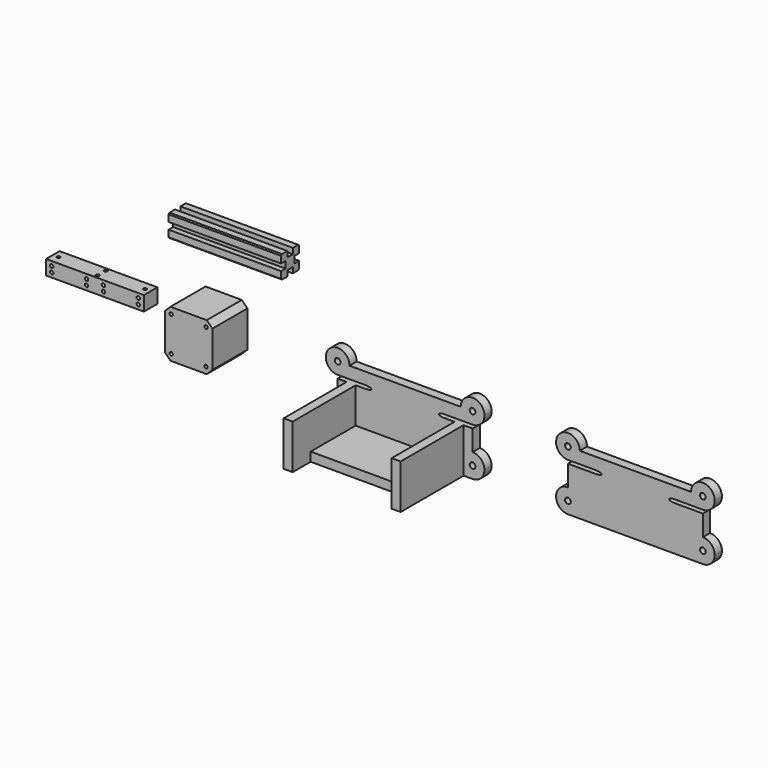
from build123d import *

# Parameters (mm, degrees)
F0_W      = 87
F0_H      = 13
F1_DEPTH  = 15
F3_DEPTH  = 25
F5_DEPTH  = 25
F7_DEPTH  = 39
F8_SIZE   = 5
F9_W      = 20
F9_H      = 20
F10_DEPTH = 100
F11_SIZE  = 1
F12_W     = 3
F12_H     = 5
F13_DEPTH = 148.2
F14_W     = 2.55
F14_H     = 15.5
F14_H_2   = 3
F15_DEPTH = 8
F18_DEPTH = 70
F19_W     = 88
F19_H     = 8
F20_DEPTH = 20


with BuildPart() as f1:
    # F0 (on Front) → F1 (new body)
    with BuildSketch(Plane.XZ):
        with Locations((-28.7405982092, 21.2712910548)):
            Rectangle(F0_W, F0_H)
    extrude(amount=F1_DEPTH)

    # F2 (on face) → F3 (cut)
    with BuildSketch(Plane.XZ.offset(15)):
        with BuildLine():
            ThreePointArc((-65.7405982092, 23.7712910548), (-66.1799380374, 24.8319512266), (-67.2405982092, 25.2712910548))
            Line((-67.2405982092, 25.2712910548), (-67.2405982092, 23.7712910548))
            Line((-67.2405982092, 23.7712910548), (-67.2405982092, 22.2712910548))
            ThreePointArc((-67.2405982092, 22.2712910548), (-66.1799380374, 22.710630883), (-65.7405982092, 23.7712910548))
        make_face()
        with BuildLine():
            Line((-67.2405982092, 23.7712910548), (-67.2405982092, 25.2712910548))
            ThreePointArc((-67.2405982092, 25.2712910548), (-68.7405982092, 23.7712910548), (-67.2405982092, 22.2712910548))
            Line((-67.2405982092, 22.2712910548), (-67.2405982092, 23.7712910548))
        make_face()
        with BuildLine():
            ThreePointArc((-67.2405982092, 20.2712910548), (-68.7405982092, 18.7712910548), (-67.2405982092, 17.2712910548))
            Line((-67.2405982092, 17.2712910548), (-67.2405982092, 18.7712910548))
            Line((-67.2405982092, 18.7712910548), (-67.2405982092, 20.2712910548))
        make_face()
        with BuildLine():
            Line((-67.2405982092, 18.7712910548), (-67.2405982092, 17.2712910548))
            ThreePointArc((-67.2405982092, 17.2712910548), (-66.1799380374, 17.710630883), (-65.7405982092, 18.7712910548))
            ThreePointArc((-65.7405982092, 18.7712910548), (-66.1799380374, 19.8319512266), (-67.2405982092, 20.2712910548))
            Line((-67.2405982092, 20.2712910548), (-67.2405982092, 18.7712910548))
        make_face()
        with BuildLine():
            Line((-34.7405982092, 23.7712910548), (-36.2405982092, 23.7712910548))
            Line((-36.2405982092, 23.7712910548), (-36.2405982092, 22.2712910548))
            ThreePointArc((-36.2405982092, 22.2712910548), (-35.1799380374, 22.710630883), (-34.7405982092, 23.7712910548))
        make_face()
        with BuildLine():
            Line((-36.2405982092, 23.7712910548), (-36.2405982092, 25.2712910548))
            ThreePointArc((-36.2405982092, 25.2712910548), (-37.7405982092, 23.7712910548), (-36.2405982092, 22.2712910548))
            Line((-36.2405982092, 22.2712910548), (-36.2405982092, 23.7712910548))
        make_face()
        with BuildLine():
            ThreePointArc((-34.7405982092, 23.7712910548), (-35.1799380374, 24.8319512266), (-36.2405982092, 25.2712910548))
            Line((-36.2405982092, 25.2712910548), (-36.2405982092, 23.7712910548))
            Line((-36.2405982092, 23.7712910548), (-34.7405982092, 23.7712910548))
        make_face()
        with BuildLine():
            ThreePointArc((-34.7405982092, 18.7712910548), (-35.1799380374, 19.8319512266), (-36.2405982092, 20.2712910548))
            ThreePointArc((-36.2405982092, 20.2712910548), (-37.301258381, 17.710630883), (-34.7405982092, 18.7712910548))
        make_face()
        with BuildLine():
            ThreePointArc((-19.7405982092, 23.7712910548), (-21.2405982092, 25.2712910548), (-22.7405982092, 23.7712910548))
            Line((-22.7405982092, 23.7712910548), (-21.2405982092, 23.7712910548))
            Line((-21.2405982092, 23.7712910548), (-21.2405982092, 22.2712910548))
            ThreePointArc((-21.2405982092, 22.2712910548), (-20.1799380374, 22.710630883), (-19.7405982092, 23.7712910548))
        make_face()
        with BuildLine():
            Line((-21.2405982092, 23.7712910548), (-22.7405982092, 23.7712910548))
            ThreePointArc((-22.7405982092, 23.7712910548), (-22.301258381, 22.710630883), (-21.2405982092, 22.2712910548))
            Line((-21.2405982092, 22.2712910548), (-21.2405982092, 23.7712910548))
        make_face()
        with BuildLine():
            Line((-21.2405982092, 18.7712910548), (-21.2405982092, 20.2712910548))
            ThreePointArc((-21.2405982092, 20.2712910548), (-22.301258381, 17.710630883), (-19.7405982092, 18.7712910548))
            Line((-19.7405982092, 18.7712910548), (-21.2405982092, 18.7712910548))
        make_face()
        with BuildLine():
            ThreePointArc((-19.7405982092, 18.7712910548), (-20.1799380374, 19.8319512266), (-21.2405982092, 20.2712910548))
            Line((-21.2405982092, 20.2712910548), (-21.2405982092, 18.7712910548))
            Line((-21.2405982092, 18.7712910548), (-19.7405982092, 18.7712910548))
        make_face()
        with BuildLine():
            Line((9.7594017908, 18.7712910548), (8.2594017908, 18.7712910548))
            ThreePointArc((8.2594017908, 18.7712910548), (9.7594017908, 17.2712910548), (11.2594017908, 18.7712910548))
            ThreePointArc((11.2594017908, 18.7712910548), (10.8200619626, 19.8319512266), (9.7594017908, 20.2712910548))
            Line((9.7594017908, 20.2712910548), (9.7594017908, 18.7712910548))
        make_face()
        with BuildLine():
            ThreePointArc((9.7594017908, 20.2712910548), (8.698741619, 19.8319512266), (8.2594017908, 18.7712910548))
            Line((8.2594017908, 18.7712910548), (9.7594017908, 18.7712910548))
            Line((9.7594017908, 18.7712910548), (9.7594017908, 20.2712910548))
        make_face()
        with BuildLine():
            ThreePointArc((11.2594017908, 23.7712910548), (8.698741619, 24.8319512266), (9.7594017908, 22.2712910548))
            ThreePointArc((9.7594017908, 22.2712910548), (10.8200619626, 22.710630883), (11.2594017908, 23.7712910548))
        make_face()
    extrude(amount=-F3_DEPTH, mode=Mode.SUBTRACT)

    # F4 (on face) → F5 (cut)
    with BuildSketch(Plane.XY.offset(27.7712910548)):
        with BuildLine():
            Line((-68.7405982092, -7.5), (-67.2405982092, -7.5))
            Line((-67.2405982092, -7.5), (-65.7405982092, -7.5))
            ThreePointArc((-65.7405982092, -7.5), (-67.2405982092, -6), (-68.7405982092, -7.5))
        make_face()
        with BuildLine():
            Line((-65.7405982092, -7.5), (-67.2405982092, -7.5))
            Line((-67.2405982092, -7.5), (-68.7405982092, -7.5))
            ThreePointArc((-68.7405982092, -7.5), (-67.2405982092, -9), (-65.7405982092, -7.5))
        make_face()
        with BuildLine():
            ThreePointArc((-28.7405982092, -1.5), (-30.2405982092, -3), (-28.7405982092, -4.5))
            Line((-28.7405982092, -4.5), (-28.7405982092, -3))
            Line((-28.7405982092, -3), (-28.7405982092, -1.5))
        make_face()
        with BuildLine():
            Line((-28.7405982092, -3), (-28.7405982092, -4.5))
            ThreePointArc((-28.7405982092, -4.5), (-27.6799380374, -4.0606601718), (-27.2405982092, -3))
            ThreePointArc((-27.2405982092, -3), (-27.6799380374, -1.9393398282), (-28.7405982092, -1.5))
            Line((-28.7405982092, -1.5), (-28.7405982092, -3))
        make_face()
        with BuildLine():
            ThreePointArc((11.2594017908, -7.5), (9.7594017908, -6), (8.2594017908, -7.5))
            Line((8.2594017908, -7.5), (9.7594017908, -7.5))
            Line((9.7594017908, -7.5), (11.2594017908, -7.5))
        make_face()
        with BuildLine():
            Line((9.7594017908, -7.5), (8.2594017908, -7.5))
            ThreePointArc((8.2594017908, -7.5), (9.7594017908, -9), (11.2594017908, -7.5))
            Line((11.2594017908, -7.5), (9.7594017908, -7.5))
        make_face()
        with BuildLine():
            ThreePointArc((-27.2405982092, -12), (-27.6799380374, -10.9393398282), (-28.7405982092, -10.5))
            Line((-28.7405982092, -10.5), (-28.7405982092, -12))
            Line((-28.7405982092, -12), (-28.7405982092, -13.5))
            ThreePointArc((-28.7405982092, -13.5), (-27.6799380374, -13.0606601718), (-27.2405982092, -12))
        make_face()
        with BuildLine():
            Line((-28.7405982092, -12), (-28.7405982092, -10.5))
            ThreePointArc((-28.7405982092, -10.5), (-30.2405982092, -12), (-28.7405982092, -13.5))
            Line((-28.7405982092, -13.5), (-28.7405982092, -12))
        make_face()
    extrude(amount=-F5_DEPTH, mode=Mode.SUBTRACT)


with BuildPart() as f7:
    # F6 (on Front) → F7 (new body)
    with BuildSketch(Plane.XZ):
        with BuildLine():
            Line((58.2019463181, 42.3), (52.5519463181, 42.3))
            Line((52.5519463181, 42.3), (52.5519463181, 36.65))
            Line((52.5519463181, 36.65), (56.7019463181, 36.65))
            ThreePointArc((56.7019463181, 36.65), (57.1412861464, 37.7106601718), (58.2019463181, 38.15))
            Line((58.2019463181, 38.15), (58.2019463181, 42.3))
        make_face()
        with BuildLine():
            Line((94.8519463181, 42.3), (58.2019463181, 42.3))
            Line((58.2019463181, 42.3), (58.2019463181, 38.15))
            ThreePointArc((58.2019463181, 38.15), (59.2626064899, 37.7106601718), (59.7019463181, 36.65))
            Line((59.7019463181, 36.65), (87.7019463181, 36.65))
            ThreePointArc((87.7019463181, 36.65), (89.2019463181, 38.15), (90.7019463181, 36.65))
            Line((90.7019463181, 36.65), (94.8519463181, 36.65))
            Line((94.8519463181, 36.65), (94.8519463181, 42.3))
        make_face()
        with BuildLine():
            Line((56.7019463181, 36.65), (52.5519463181, 36.65))
            Line((52.5519463181, 36.65), (52.5519463181, 0))
            Line((52.5519463181, 0), (94.8519463181, 0))
            Line((94.8519463181, 0), (94.8519463181, 36.65))
            Line((94.8519463181, 36.65), (90.7019463181, 36.65))
            ThreePointArc((90.7019463181, 36.65), (90.2626064899, 35.5893398282), (89.2019463181, 35.15))
            Line((89.2019463181, 35.15), (89.2019463181, 7.15))
            ThreePointArc((89.2019463181, 7.15), (90.2626064899, 6.7106601718), (90.7019463181, 5.65))
            ThreePointArc((90.7019463181, 5.65), (89.2019463181, 4.15), (87.7019463181, 5.65))
            Line((87.7019463181, 5.65), (59.7019463181, 5.65))
            ThreePointArc((59.7019463181, 5.65), (57.1412861464, 4.5893398282), (58.2019463181, 7.15))
            Line((58.2019463181, 7.15), (58.2019463181, 35.15))
            ThreePointArc((58.2019463181, 35.15), (57.1412861464, 35.5893398282), (56.7019463181, 36.65))
        make_face()
        with BuildLine():
            Line((87.7019463181, 36.65), (59.7019463181, 36.65))
            ThreePointArc((59.7019463181, 36.65), (59.2626064899, 35.5893398282), (58.2019463181, 35.15))
            Line((58.2019463181, 35.15), (58.2019463181, 7.15))
            ThreePointArc((58.2019463181, 7.15), (59.2626064899, 6.7106601718), (59.7019463181, 5.65))
            Line((59.7019463181, 5.65), (87.7019463181, 5.65))
            ThreePointArc((87.7019463181, 5.65), (88.1412861464, 6.7106601718), (89.2019463181, 7.15))
            Line((89.2019463181, 7.15), (89.2019463181, 35.15))
            ThreePointArc((89.2019463181, 35.15), (88.1412861464, 35.5893398282), (87.7019463181, 36.65))
        make_face()
    extrude(amount=F7_DEPTH)

    # F8
    f8_edges = [f7.edges().sort_by_distance(p)[0] for p in [
        (52.551946, -19.5, 42.3),
        (94.851946, -19.5, 42.3),
        (52.551946, -19.5, 0),
        (94.851946, -19.5, 0),
    ]]
    chamfer(f8_edges, length=F8_SIZE)


with BuildPart() as f10:
    # F9 (on Right) → F10 (new body)
    with BuildSketch(Plane.YZ):
        with Locations((41.0009028763, 58.4589114785)):
            Rectangle(F9_W, F9_H)
    extrude(amount=F10_DEPTH)

    # F11
    f11_edges = [f10.edges().sort_by_distance(p)[0] for p in [
        (50, 31.000903, 68.458911),
        (50, 51.000903, 68.458911),
        (50, 31.000903, 48.458911),
        (50, 51.000903, 48.458911),
    ]]
    chamfer(f11_edges, length=F11_SIZE)

    # F12 (on face) → F13 (cut)
    with BuildSketch(Plane(origin=(0, 0, 0), x_dir=(0, -1, 0), z_dir=(-1, 0, 0))):
        with Locations((-42.5009028763, 50.9589114785)):
            Rectangle(F12_W, F12_H)
        with Locations((-39.5009028763, 50.9589114785)):
            Rectangle(F12_W, F12_H)
        with Locations((-42.5009028763, 65.9589114785)):
            Rectangle(F12_W, F12_H)
        with Locations((-39.5009028763, 65.9589114785)):
            Rectangle(F12_W, F12_H)
        Polygon((-46.0009028763, 61.4589114785), (-51.0009028763, 61.4589114785), (-51.0009028763, 58.4589114785), (-51.0009028763, 55.4589114785), (-46.0009028763, 55.4589114785), align=None)
        Polygon((-31.0009028763, 61.4589114785), (-36.0009028763, 61.4589114785), (-36.0009028763, 58.4589114785), (-36.0009028763, 55.4589114785), (-31.0009028763, 55.4589114785), align=None)
    extrude(amount=-F13_DEPTH, mode=Mode.SUBTRACT)


with BuildPart() as f15:
    # F14 (on Front) → F15 (new body)
    with BuildSketch(Plane.XZ):
        with BuildLine():
            ThreePointArc((178.9015343745, 27.2655571997), (181.4515343745, 29.8155571997), (184.0015343745, 27.2655571997))
            Line((184.0015343745, 27.2655571997), (192.0015343745, 27.2655571997))
            ThreePointArc((192.0015343745, 27.2655571997), (181.4515343745, 37.8155571997), (170.9015343745, 27.2655571997))
            Line((170.9015343745, 27.2655571997), (178.9015343745, 27.2655571997))
        make_face()
        with BuildLine():
            Line((192.0015343745, 27.2655571997), (184.0015343745, 27.2655571997))
            ThreePointArc((184.0015343745, 27.2655571997), (183.2546566665, 25.4624349077), (181.4515343745, 24.7155571997))
            Line((181.4515343745, 24.7155571997), (181.4515343745, 16.7155571997))
            ThreePointArc((181.4515343745, 16.7155571997), (188.911510916, 19.8055806582), (192.0015343745, 27.2655571997))
        make_face()
        with BuildLine():
            Line((181.4515343745, 16.7155571997), (181.4515343745, 24.7155571997))
            ThreePointArc((181.4515343745, 24.7155571997), (179.6484120825, 25.4624349077), (178.9015343745, 27.2655571997))
            Line((178.9015343745, 27.2655571997), (170.9015343745, 27.2655571997))
            ThreePointArc((170.9015343745, 27.2655571997), (173.991557833, 19.8055806582), (181.4515343745, 16.7155571997))
        make_face()
        with BuildLine():
            Line((241.4515343745, 27.2655571997), (192.0015343745, 27.2655571997))
            ThreePointArc((192.0015343745, 27.2655571997), (188.911510916, 19.8055806582), (181.4515343745, 16.7155571997))
            Line((181.4515343745, 16.7155571997), (206.4515343745, 16.7155571997))
            Line((206.4515343745, 16.7155571997), (211.4515343745, 16.7155571997))
            Line((211.4515343745, 16.7155571997), (241.4515343745, 16.7155571997))
            Line((241.4515343745, 16.7155571997), (241.4515343745, 27.2655571997))
        make_face()
        with BuildLine():
            Line((282.7265343745, 27.2655571997), (241.4515343745, 27.2655571997))
            Line((241.4515343745, 27.2655571997), (241.4515343745, 16.7155571997))
            Line((241.4515343745, 16.7155571997), (276.4515343745, 16.7155571997))
            Line((276.4515343745, 16.7155571997), (290.9015343745, 16.7155571997))
            Line((290.9015343745, 16.7155571997), (301.4515343745, 16.7155571997))
            ThreePointArc((301.4515343745, 16.7155571997), (293.991557833, 19.8055806582), (290.9015343745, 27.2655571997))
            Line((290.9015343745, 27.2655571997), (282.7265343745, 27.2655571997))
        make_face()
        Polygon((184.0015343745, 13.7155571997), (181.4515343745, 13.7155571997), (181.4515343745, -1.7844428003), (206.4515343745, -1.7844428003), (211.4515343745, -1.7844428003), (211.4515343745, 13.7155571997), (206.4515343745, 13.7155571997), (192.0015343745, 13.7155571997), align=None)
        with BuildLine():
            Line((211.4515343745, 16.7155571997), (206.4515343745, 16.7155571997))
            add(Edge.make_bspline(
                [(211.4515343745, 15.2155571997), (211.4515343745, 16.7155571997), (206.4515343745, 16.7155571997)],
                knots=[0, 0, 0, 1.5707963268, 1.5707963268, 1.5707963268], degree=2, weights=[1, 0.7071067812, 1]))
            Line((211.4515343745, 15.2155571997), (211.4515343745, 16.7155571997))
        make_face()
        Polygon((241.4515343745, 13.7155571997), (241.4515343745, 16.7155571997), (211.4515343745, 16.7155571997), (211.4515343745, 15.2155571997), (211.4515343745, 13.7155571997), align=None)
        with BuildLine():
            Line((276.4515343745, 16.7155571997), (241.4515343745, 16.7155571997))
            Line((241.4515343745, 16.7155571997), (241.4515343745, 13.7155571997))
            Line((241.4515343745, 13.7155571997), (276.4515343664, 13.7155571997))
            add(Edge.make_bspline(
                [(271.4515343745, 15.2155571997), (271.4515343745, 13.7155572022), (276.4515343664, 13.7155571997)],
                knots=[0, 0, 0, 1.5707963252, 1.5707963252, 1.5707963252], degree=2, weights=[1, 0.7071067818, 1]))
            add(Edge.make_bspline(
                [(276.4515343745, 16.7155571997), (271.4515343745, 16.7155571997), (271.4515343745, 15.2155571997)],
                knots=[4.7123889804, 4.7123889804, 4.7123889804, 6.2831853072, 6.2831853072, 6.2831853072], degree=2, weights=[1, 0.7071067812, 1]))
        make_face()
        with BuildLine():
            Line((206.4515343745, -1.7844428003), (181.4515343745, -1.7844428003))
            Line((181.4515343745, -1.7844428003), (181.4515343745, -4.7844428003))
            Line((181.4515343745, -4.7844428003), (206.4515343745, -4.7844428003))
            add(Edge.make_bspline(
                [(206.4515343745, -1.7844428003), (201.4515343745, -1.7844428003), (201.4515343745, -3.2844428003), (201.4515343745, -4.7844428003), (206.4515343745, -4.7844428003)],
                knots=[1.5707963268, 1.5707963268, 1.5707963268, 3.1415926536, 3.1415926536, 4.7123889804, 4.7123889804, 4.7123889804], degree=2, weights=[1, 0.7071067812, 1, 0.7071067812, 1]))
        make_face()
        with BuildLine():
            Line((211.4515343745, 13.7155571997), (211.4515343745, 15.2155571997))
            add(Edge.make_bspline(
                [(206.4515343745, 13.7155571997), (211.4515343745, 13.7155571997), (211.4515343745, 15.2155571997)],
                knots=[4.7123889804, 4.7123889804, 4.7123889804, 6.2831853072, 6.2831853072, 6.2831853072], degree=2, weights=[1, 0.7071067812, 1]))
            Line((206.4515343745, 13.7155571997), (211.4515343745, 13.7155571997))
        make_face()
        with BuildLine():
            ThreePointArc((312.0015343745, 27.2655571997), (301.4515343745, 37.8155571997), (290.9015343745, 27.2655571997))
            ThreePointArc((290.9015343745, 27.2655571997), (293.991557833, 19.8055806582), (301.4515343745, 16.7155571997))
            ThreePointArc((301.4515343745, 16.7155571997), (308.911510916, 19.8055806582), (312.0015343745, 27.2655571997))
        make_face()
        with BuildLine():
            ThreePointArc((304.0015343745, 27.2655571997), (303.2546566665, 25.4624349077), (301.4515343745, 24.7155571997))
            ThreePointArc((301.4515343745, 24.7155571997), (299.6484120825, 29.0686794917), (304.0015343745, 27.2655571997))
        make_face(mode=Mode.SUBTRACT)
        Polygon((241.4515343745, 5.9655571997), (241.4515343745, 13.7155571997), (211.4515343745, 13.7155571997), (211.4515343745, -1.7844428003), (241.4515343745, -1.7844428003), align=None)
        Polygon((276.4515343664, 13.7155571997), (241.4515343745, 13.7155571997), (241.4515343745, 5.9655571997), (241.4515343745, -1.7844428003), (276.4515343745, -1.7844428003), (290.9015343745, -1.7844428003), (298.9015343745, -1.7844428003), (298.9015343745, 13.7155571997), (290.9015343745, 13.7155571997), align=None)
        with BuildLine():
            ThreePointArc((192.0015343745, -15.3344428003), (188.911510916, -7.8744662588), (181.4515343745, -4.7844428003))
            Line((181.4515343745, -4.7844428003), (181.4515343745, -12.7844428003))
            ThreePointArc((181.4515343745, -12.7844428003), (183.2546566665, -13.5313205083), (184.0015343745, -15.3344428003))
            Line((184.0015343745, -15.3344428003), (192.0015343745, -15.3344428003))
        make_face()
        with BuildLine():
            Line((206.4515343745, -4.7844428003), (181.4515343745, -4.7844428003))
            ThreePointArc((181.4515343745, -4.7844428003), (188.911510916, -7.8744662588), (192.0015343745, -15.3344428003))
            Line((192.0015343745, -15.3344428003), (241.4515343745, -15.3344428003))
            Line((241.4515343745, -15.3344428003), (241.4515343745, -4.7844428003))
            Line((241.4515343745, -4.7844428003), (211.4515343745, -4.7844428003))
            Line((211.4515343745, -4.7844428003), (206.4515343745, -4.7844428003))
        make_face()
        with BuildLine():
            Line((181.4515343745, -12.7844428003), (181.4515343745, -4.7844428003))
            ThreePointArc((181.4515343745, -4.7844428003), (173.991557833, -7.8744662588), (170.9015343745, -15.3344428003))
            Line((170.9015343745, -15.3344428003), (178.9015343745, -15.3344428003))
            ThreePointArc((178.9015343745, -15.3344428003), (179.6484120825, -13.5313205083), (181.4515343745, -12.7844428003))
        make_face()
        with BuildLine():
            Line((211.4515343745, -1.7844428003), (206.4515343745, -1.7844428003))
            add(Edge.make_bspline(
                [(211.4515343745, -3.2844428003), (211.4515343745, -1.7844428003), (206.4515343745, -1.7844428003)],
                knots=[0, 0, 0, 1.5707963268, 1.5707963268, 1.5707963268], degree=2, weights=[1, 0.7071067812, 1]))
            Line((211.4515343745, -3.2844428003), (211.4515343745, -1.7844428003))
        make_face()
        with BuildLine():
            add(Edge.make_bspline(
                [(211.4515343745, -3.2844428003), (211.4515343745, -1.7844428003), (206.4515343745, -1.7844428003)],
                knots=[0, 0, 0, 1.5707963268, 1.5707963268, 1.5707963268], degree=2, weights=[1, 0.7071067812, 1]))
            add(Edge.make_bspline(
                [(206.4515343745, -1.7844428003), (201.4515343745, -1.7844428003), (201.4515343745, -3.2844428003), (201.4515343745, -4.7844428003), (206.4515343745, -4.7844428003)],
                knots=[1.5707963268, 1.5707963268, 1.5707963268, 3.1415926536, 3.1415926536, 4.7123889804, 4.7123889804, 4.7123889804], degree=2, weights=[1, 0.7071067812, 1, 0.7071067812, 1]))
            add(Edge.make_bspline(
                [(206.4515343745, -4.7844428003), (211.4515343745, -4.7844428003), (211.4515343745, -3.2844428003)],
                knots=[4.7123889804, 4.7123889804, 4.7123889804, 6.2831853072, 6.2831853072, 6.2831853072], degree=2, weights=[1, 0.7071067812, 1]))
        make_face()
        with BuildLine():
            ThreePointArc((181.4515343745, -25.8844428003), (188.911510916, -22.7944193418), (192.0015343745, -15.3344428003))
            Line((192.0015343745, -15.3344428003), (184.0015343745, -15.3344428003))
            ThreePointArc((184.0015343745, -15.3344428003), (183.2546566665, -17.1375650923), (181.4515343745, -17.8844428003))
            Line((181.4515343745, -17.8844428003), (181.4515343745, -25.8844428003))
        make_face()
        with BuildLine():
            Line((241.4515343745, -15.3344428003), (192.0015343745, -15.3344428003))
            ThreePointArc((192.0015343745, -15.3344428003), (188.911510916, -22.7944193418), (181.4515343745, -25.8844428003))
            Line((181.4515343745, -25.8844428003), (192.0015343745, -25.8844428003))
            Line((192.0015343745, -25.8844428003), (241.4515343745, -25.8844428003))
            Line((241.4515343745, -25.8844428003), (241.4515343745, -15.3344428003))
        make_face()
        with BuildLine():
            Line((178.9015343745, -15.3344428003), (170.9015343745, -15.3344428003))
            ThreePointArc((170.9015343745, -15.3344428003), (173.991557833, -22.7944193418), (181.4515343745, -25.8844428003))
            Line((181.4515343745, -25.8844428003), (181.4515343745, -17.8844428003))
            ThreePointArc((181.4515343745, -17.8844428003), (179.6484120825, -17.1375650923), (178.9015343745, -15.3344428003))
        make_face()
        with BuildLine():
            add(Edge.make_bspline(
                [(206.4515343745, -4.7844428003), (211.4515343745, -4.7844428003), (211.4515343745, -3.2844428003)],
                knots=[4.7123889804, 4.7123889804, 4.7123889804, 6.2831853072, 6.2831853072, 6.2831853072], degree=2, weights=[1, 0.7071067812, 1]))
            Line((206.4515343745, -4.7844428003), (211.4515343745, -4.7844428003))
            Line((211.4515343745, -4.7844428003), (211.4515343745, -3.2844428003))
        make_face()
        Polygon((241.4515343745, -1.7844428003), (211.4515343745, -1.7844428003), (211.4515343745, -3.2844428003), (211.4515343745, -4.7844428003), (241.4515343745, -4.7844428003), align=None)
        with Locations((300.1765343745, 5.9655571997)):
            Rectangle(F14_W, F14_H)
        with BuildLine():
            Line((276.4515343745, -1.7844428003), (241.4515343745, -1.7844428003))
            Line((241.4515343745, -1.7844428003), (241.4515343745, -4.7844428003))
            Line((241.4515343745, -4.7844428003), (262.8303221703, -4.7844428003))
            Line((262.8303221703, -4.7844428003), (276.4515343745, -4.7844428003))
            add(Edge.make_bspline(
                [(271.4515343745, -3.2844428003), (271.4515343745, -4.7844428003), (276.4515343745, -4.7844428003)],
                knots=[0, 0, 0, 1.5707963268, 1.5707963268, 1.5707963268], degree=2, weights=[1, 0.7071067812, 1]))
            add(Edge.make_bspline(
                [(276.4515343745, -1.7844428003), (271.4515343745, -1.7844428003), (271.4515343745, -3.2844428003)],
                knots=[4.7123889804, 4.7123889804, 4.7123889804, 6.2831853072, 6.2831853072, 6.2831853072], degree=2, weights=[1, 0.7071067812, 1]))
        make_face()
        with BuildLine():
            Line((241.4515343745, -4.7844428003), (241.4515343745, -15.3344428003))
            Line((241.4515343745, -15.3344428003), (282.7265343745, -15.3344428003))
            Line((282.7265343745, -15.3344428003), (290.7265343745, -15.3344428003))
            Line((290.7265343745, -15.3344428003), (290.9015343745, -15.3344428003))
            ThreePointArc((290.9015343745, -15.3344428003), (293.1387430262, -8.8382900927), (298.9015343745, -5.0972556866))
            Line((298.9015343745, -5.0972556866), (298.9015343745, -4.7844428003))
            Line((298.9015343745, -4.7844428003), (276.4515343745, -4.7844428003))
            Line((276.4515343745, -4.7844428003), (262.8303221703, -4.7844428003))
            Line((262.8303221703, -4.7844428003), (241.4515343745, -4.7844428003))
        make_face()
        with BuildLine():
            Line((282.7265343745, -15.3344428003), (241.4515343745, -15.3344428003))
            Line((241.4515343745, -15.3344428003), (241.4515343745, -25.8844428003))
            Line((241.4515343745, -25.8844428003), (285.4515343745, -25.8844428003))
            Line((285.4515343745, -25.8844428003), (290.9015343745, -25.8844428003))
            Line((290.9015343745, -25.8844428003), (301.4515343745, -25.8844428003))
            ThreePointArc((301.4515343745, -25.8844428003), (300.1669768727, -25.8059475644), (298.9015343745, -25.5716299139))
            ThreePointArc((298.9015343745, -25.5716299139), (293.1387430262, -21.8305955078), (290.9015343745, -15.3344428003))
            Line((290.9015343745, -15.3344428003), (290.7265343745, -15.3344428003))
            Line((290.7265343745, -15.3344428003), (282.7265343745, -15.3344428003))
        make_face()
        with Locations((300.1765343745, -3.2844428003)):
            Rectangle(F14_W, F14_H_2)
        with BuildLine():
            Line((290.9015343745, -1.7844428003), (276.4515343745, -1.7844428003))
            add(Edge.make_bspline(
                [(276.4515343745, -4.7844428003), (281.4515343745, -4.7844428003), (281.4515343745, -3.2844428003), (281.4515343745, -1.7844428003), (276.4515343745, -1.7844428003)],
                knots=[1.5707963268, 1.5707963268, 1.5707963268, 3.1415926536, 3.1415926536, 4.7123889804, 4.7123889804, 4.7123889804], degree=2, weights=[1, 0.7071067812, 1, 0.7071067812, 1]))
            Line((276.4515343745, -4.7844428003), (298.9015343745, -4.7844428003))
            Line((298.9015343745, -4.7844428003), (298.9015343745, -1.7844428003))
            Line((298.9015343745, -1.7844428003), (290.9015343745, -1.7844428003))
        make_face()
        with BuildLine():
            add(Edge.make_bspline(
                [(276.4515343745, -4.7844428003), (281.4515343745, -4.7844428003), (281.4515343745, -3.2844428003), (281.4515343745, -1.7844428003), (276.4515343745, -1.7844428003)],
                knots=[1.5707963268, 1.5707963268, 1.5707963268, 3.1415926536, 3.1415926536, 4.7123889804, 4.7123889804, 4.7123889804], degree=2, weights=[1, 0.7071067812, 1, 0.7071067812, 1]))
            add(Edge.make_bspline(
                [(276.4515343745, -1.7844428003), (271.4515343745, -1.7844428003), (271.4515343745, -3.2844428003)],
                knots=[4.7123889804, 4.7123889804, 4.7123889804, 6.2831853072, 6.2831853072, 6.2831853072], degree=2, weights=[1, 0.7071067812, 1]))
            add(Edge.make_bspline(
                [(271.4515343745, -3.2844428003), (271.4515343745, -4.7844428003), (276.4515343745, -4.7844428003)],
                knots=[0, 0, 0, 1.5707963268, 1.5707963268, 1.5707963268], degree=2, weights=[1, 0.7071067812, 1]))
        make_face()
        with BuildLine():
            Line((301.4515343745, -12.7844428003), (301.4515343745, -4.7844428003))
            ThreePointArc((301.4515343745, -4.7844428003), (300.1669768727, -4.8629380362), (298.9015343745, -5.0972556866))
            Line((298.9015343745, -5.0972556866), (298.9015343745, -15.3344428003))
            ThreePointArc((298.9015343745, -15.3344428003), (299.6484120825, -13.5313205083), (301.4515343745, -12.7844428003))
        make_face()
        with BuildLine():
            ThreePointArc((312.0015343745, -15.3344428003), (308.911510916, -7.8744662588), (301.4515343745, -4.7844428003))
            Line((301.4515343745, -4.7844428003), (301.4515343745, -12.7844428003))
            ThreePointArc((301.4515343745, -12.7844428003), (303.2546566665, -13.5313205083), (304.0015343745, -15.3344428003))
            ThreePointArc((304.0015343745, -15.3344428003), (301.4515343745, -17.8844428003), (298.9015343745, -15.3344428003))
            Line((298.9015343745, -15.3344428003), (298.9015343745, -25.5716299139))
            ThreePointArc((298.9015343745, -25.5716299139), (300.1669768727, -25.8059475644), (301.4515343745, -25.8844428003))
            ThreePointArc((301.4515343745, -25.8844428003), (308.911510916, -22.7944193418), (312.0015343745, -15.3344428003))
        make_face()
        with BuildLine():
            ThreePointArc((298.9015343745, -5.0972556866), (300.1669768727, -4.8629380362), (301.4515343745, -4.7844428003))
            Line((301.4515343745, -4.7844428003), (298.9015343745, -4.7844428003))
            Line((298.9015343745, -4.7844428003), (298.9015343745, -5.0972556866))
        make_face()
        with BuildLine():
            Line((298.9015343745, -15.3344428003), (298.9015343745, -5.0972556866))
            ThreePointArc((298.9015343745, -5.0972556866), (293.1387430262, -8.8382900927), (290.9015343745, -15.3344428003))
            Line((290.9015343745, -15.3344428003), (298.9015343745, -15.3344428003))
        make_face()
        with BuildLine():
            Line((298.9015343745, -15.3344428003), (290.9015343745, -15.3344428003))
            ThreePointArc((290.9015343745, -15.3344428003), (293.1387430262, -21.8305955078), (298.9015343745, -25.5716299139))
            Line((298.9015343745, -25.5716299139), (298.9015343745, -15.3344428003))
        make_face()
    extrude(amount=F15_DEPTH)


with BuildPart() as f16_1:
    # F16: copy of F15
    add(f15.part.moved(Location((204.8, 0, 0))))


with BuildPart() as f15_1:
    add(f15.part)

    # F17 (on face) → F18 (join)
    with BuildSketch(Plane.XZ.offset(8)):
        Polygon((189.4515343745, 13.7155571997), (189.4515343745, -25.8844428003), (197.4515343745, -25.8844428003), (197.4515343745, -17.8844428003), (197.4515343745, 13.7155571997), align=None)
        Polygon((197.4515343745, -17.8844428003), (197.4515343745, -25.8844428003), (241.4515343745, -25.8844428003), (285.4515343745, -25.8844428003), (285.4515343745, -17.8844428003), align=None)
        Polygon((285.4515343745, -17.8844428003), (285.4515343745, -25.8844428003), (293.4515343745, -25.8844428003), (293.4515343745, 13.7155571997), (285.4515343745, 13.7155571997), align=None)
    extrude(amount=F18_DEPTH)

    # F19 (on face) → F20 (cut)
    with BuildSketch(Plane.XZ.offset(78)):
        with Locations((241.4515343745, -21.8844428003)):
            Rectangle(F19_W, F19_H)
    extrude(amount=-F20_DEPTH, mode=Mode.SUBTRACT)


solid = Compound([f1.part, f7.part, f10.part, f16_1.part, f15_1.part])
